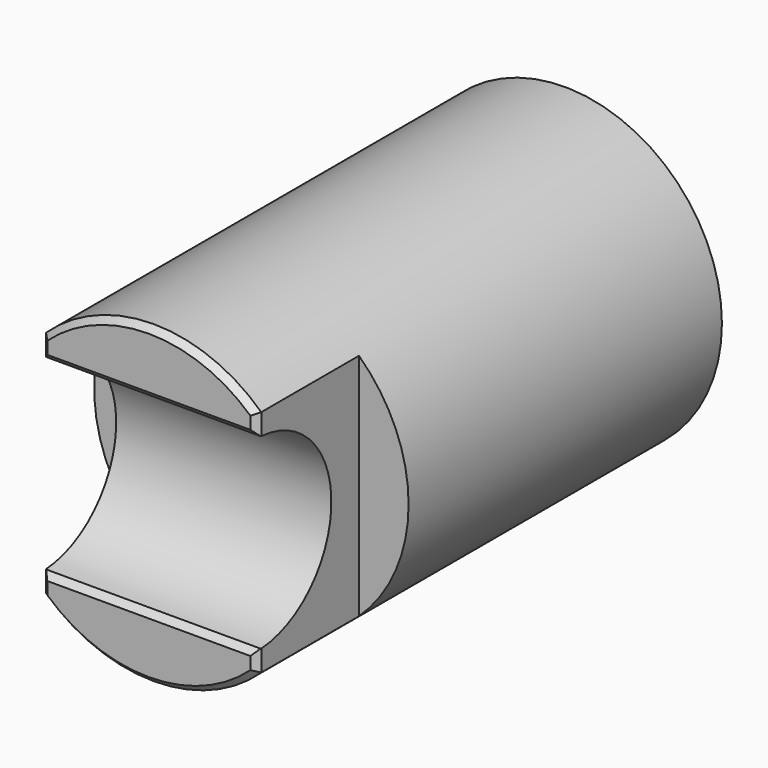
from build123d import *

# Parameters (mm, degrees)
F0_R          = 13.005
F1_DEPTH      = 43
F2_R          = 7.75
F3_DEPTH      = 13.006
F3_DEPTH_BACK = 25
F4_W          = 7.1834153318
F4_H          = 12.5
F5_DEPTH      = 12.5
F6_T1_DEPTH   = 4.3042999791
F6_T3_DEPTH   = 20.2979349857
F6_T5_DEPTH   = 4.3042999791
F6_T8_ANGLE   = 97.7035470752
F6_T10_ANGLE  = 97.7035470752


# Not quite as in the source:
# - a fillet or chamfer that OpenCascade refuses, or shapes differently, is made with other operations: its cross-section is extruded or revolved along the edge and cut away or added


with BuildPart() as f1:
    # F0 (on Front) → F1 (new body)
    with BuildSketch(Plane.XZ):
        Circle(F0_R)
    extrude(amount=-F1_DEPTH)

    # F2 (on Right) → F3 (cut, two sides)
    with BuildSketch(Plane.YZ) as f3_sk:
        Circle(F2_R)
    extrude(amount=-F3_DEPTH, mode=Mode.SUBTRACT)
    extrude(f3_sk.sketch, amount=F3_DEPTH_BACK, mode=Mode.SUBTRACT)

    # F4 (on Top) → F5 (cut, symmetric)
    with BuildSketch(Plane.XY):
        with Locations((12.4917076659, 4.3530291878)):
            Rectangle(F4_W, F4_H)
        with Locations((-12.4917076659, 4.3530291878)):
            Rectangle(F4_W, F4_H)
    extrude(amount=F5_DEPTH, both=True, mode=Mode.SUBTRACT)

    # F6: chamfer of 0.5 on 8 edges, made by hand

    # F6_s2 → F6_t1 (cut)
    with BuildSketch(Plane.XY.offset(6.464158506)):
        Polygon((-8.4, 0), (-8.9, 0.5), (-8.9, 0), align=None)
        Polygon((8.9, 0.5), (8.4, 0), (8.9, 0), align=None)
    extrude(amount=F6_T1_DEPTH, mode=Mode.SUBTRACT)

    # F6_s4 → F6_t3 (cut)
    with BuildSketch(Plane.YZ.offset(-10.1489674928)):
        with BuildLine():
            Line((0, 8.234834546), (0.4696969697, 7.7357536644))
            ThreePointArc((0.4696969697, 7.7357536644), (0.2420339134, 7.7462196964), (0, 7.75))
            Line((0, 7.75), (0, 8.234834546))
        make_face()
        with BuildLine():
            Line((0, -8.234834546), (0.4696969697, -7.7357536644))
            ThreePointArc((0.4696969697, -7.7357536644), (0.2420339134, -7.7462196964), (0, -7.75))
            Line((0, -7.75), (0, -8.234834546))
        make_face()
    extrude(amount=F6_T3_DEPTH, mode=Mode.SUBTRACT)

    # F6_s6 → F6_t5 (cut)
    with BuildSketch(Plane.XY.offset(-10.7684584851)):
        Polygon((-8.9, 0.5), (-8.4, 0), (-8.9, 0), align=None)
        Polygon((8.9, 0.5), (8.4, 0), (8.9, 0), align=None)
    extrude(amount=F6_T5_DEPTH, mode=Mode.SUBTRACT)

    # F6_s7 → F6_t8 (revolve, cut)
    with BuildSketch(Plane(origin=(0, 0, 0), x_dir=(0, 1, 0), z_dir=(0.6580092951, 0, -0.7530098057))):
        Polygon((0.5, 13.005), (0, 12.505), (0, 13.005), align=None)
    revolve(axis=Axis((0, 0, 0), (0, -1, 0)), revolution_arc=F6_T8_ANGLE, mode=Mode.SUBTRACT)

    # F6_s9 → F6_t10 (revolve, cut)
    with BuildSketch(Plane(origin=(0, 0, 0), x_dir=(0, 1, 0), z_dir=(-0.6580092951, 0, 0.7530098057))):
        Polygon((0.5, 13.005), (0, 12.505), (0, 13.005), align=None)
    revolve(axis=Axis((0, 0, 0), (0, -1, 0)), revolution_arc=F6_T10_ANGLE, mode=Mode.SUBTRACT)


solid = f1.part
